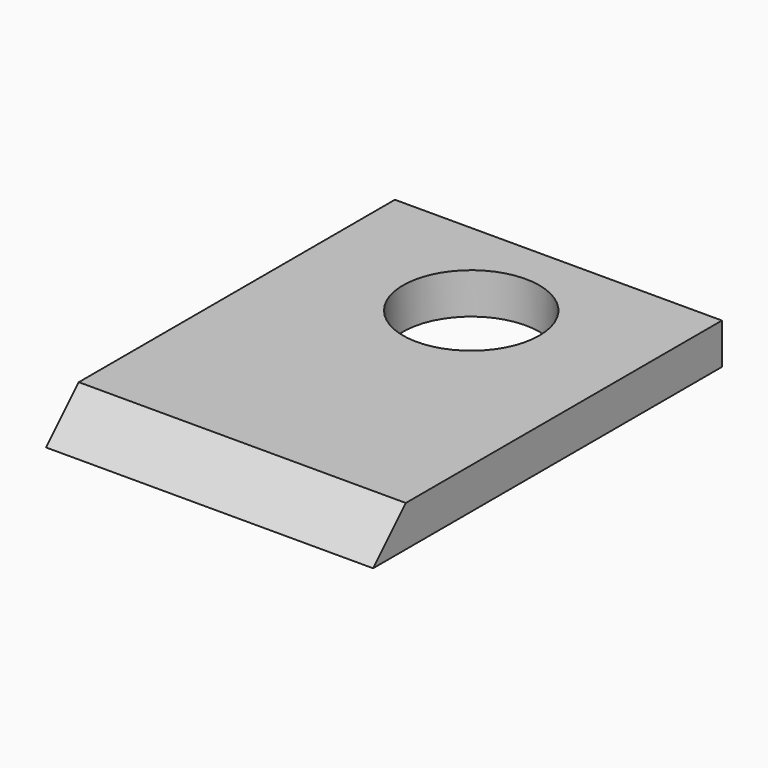
from build123d import *

# Parameters (mm, degrees)
F0_W     = 76.2
F0_H     = 101.6
F1_DEPTH = 9.525
F2_SIZE  = 9.52499
F3_R     = 15.875
F4_DEPTH = 9.525


# Not quite as in the source:
# - a fillet or chamfer is up to 0.001 mm smaller than in the source, because OpenCascade refuses the exact size


with BuildPart() as f1:
    # F0 (on Top) → F1 (new body)
    with BuildSketch(Plane.XY):
        Rectangle(F0_W, F0_H)
    extrude(amount=F1_DEPTH)

    # F2 (size 9.525 in the source; OpenCascade refuses exactly that, so slightly less here)
    f2_edges = [f1.edges().sort_by_distance(p)[0] for p in [
        (0, -50.8, 9.525),
    ]]
    chamfer(f2_edges, length=F2_SIZE)

    # F3 (on face) → F4 (cut)
    with BuildSketch(Plane(origin=(0, 0, 0), x_dir=(1, 0, 0), z_dir=(0, 0, -1))):
        with Locations((0, -25.4)):
            Circle(F3_R)
    extrude(amount=-F4_DEPTH, mode=Mode.SUBTRACT)


solid = f1.part
